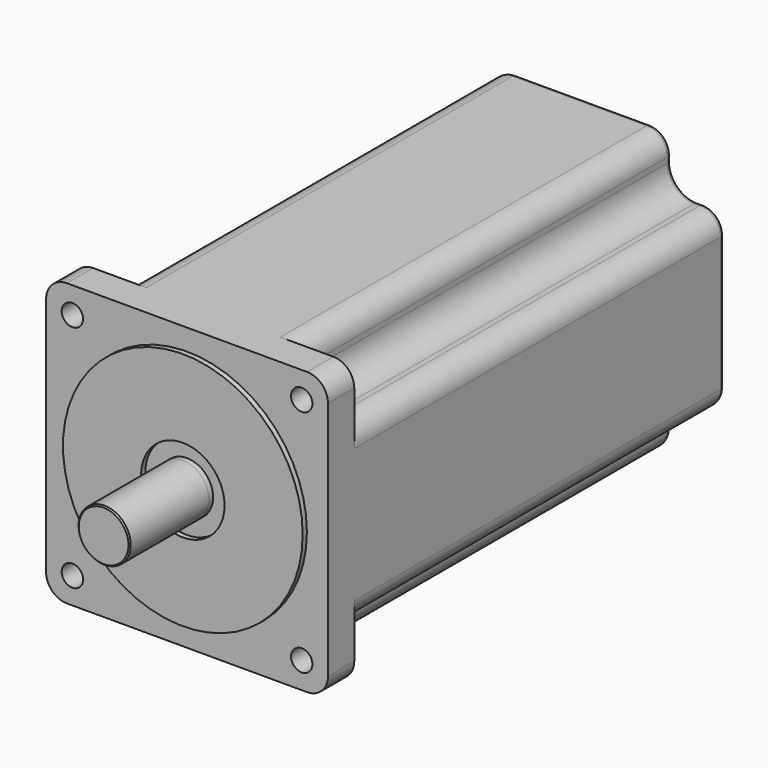
from build123d import *

# Parameters (mm, degrees)
F0_R         = 3.2512
F1_DEPTH     = 10.0076
F2_R         = 36.4998
F3_DEPTH     = 1.6002
F4_R         = 7.9375
F5_DEPTH     = 31.75
F6_SIZE      = 0.381
F7_R         = 12.7
F7_R_2       = 7.9375
F8_DEPTH     = 1.6002
F10_DEPTH    = 140.9954
F11_T1_DEPTH = 156.8704
F12_R        = 1.6002
F13_R        = 4.826
F14_DEPTH    = 12.7
F14_TAPER    = 1


# Not quite as in the source:
# - a fillet or chamfer that OpenCascade refuses, or shapes differently, is made with other operations: its cross-section is extruded or revolved along the edge and cut away or added


with BuildPart() as f1:
    # F0 (on Front) → F1 (new body)
    with BuildSketch(Plane.XZ):
        with BuildLine():
            ThreePointArc((42.926, 36.576), (41.0661280605, 41.0661280605), (36.576, 42.926))
            Line((36.576, 42.926), (-36.576, 42.926))
            ThreePointArc((-36.576, 42.926), (-41.0661280605, 41.0661280605), (-42.926, 36.576))
            Line((-42.926, 36.576), (-42.926, -36.576))
            ThreePointArc((-42.926, -36.576), (-41.0661280605, -41.0661280605), (-36.576, -42.926))
            Line((-36.576, -42.926), (36.576, -42.926))
            ThreePointArc((36.576, -42.926), (41.0661280605, -41.0661280605), (42.926, -36.576))
            Line((42.926, -36.576), (42.926, 36.576))
        make_face()
        with Locations((-34.925, -34.925)):
            Circle(F0_R, mode=Mode.SUBTRACT)
        with Locations((34.925, -34.925)):
            Circle(F0_R, mode=Mode.SUBTRACT)
        with Locations((-34.925, 34.925)):
            Circle(F0_R, mode=Mode.SUBTRACT)
        with Locations((34.925, 34.925)):
            Circle(F0_R, mode=Mode.SUBTRACT)
    extrude(amount=-F1_DEPTH)

    # F2 (on Front) → F3 (join)
    with BuildSketch(Plane.XZ):
        Circle(F2_R)
    extrude(amount=F3_DEPTH)

    # F4 (on Front) → F5 (join)
    with BuildSketch(Plane.XZ):
        Circle(F4_R)
    extrude(amount=F5_DEPTH)

    # F6
    f6_edges = [f1.edges().sort_by_distance(p)[0] for p in [
        (-7.9375, -31.75, 0),
    ]]
    chamfer(f6_edges, length=F6_SIZE)

    # F7 (on face) → F8 (cut)
    with BuildSketch(Plane.XZ.offset(1.6002)):
        Circle(F7_R)
        Circle(F7_R_2, mode=Mode.SUBTRACT)
    extrude(amount=-F8_DEPTH, mode=Mode.SUBTRACT)

    # F9 (on face) → F10 (join)
    with BuildSketch(Plane(origin=(0, 10.0076, 0), x_dir=(-1, 0, 0), z_dir=(0, 1, 0))):
        with BuildLine():
            ThreePointArc((-26.7554344057, 34.925), (-29.1482447689, 29.1482447689), (-34.925, 26.7554344057))
            Line((-34.925, 26.7554344057), (-42.926, 26.7554344057))
            Line((-42.926, 26.7554344057), (-42.926, -26.7554344057))
            Line((-42.926, -26.7554344057), (-34.925, -26.7554344057))
            ThreePointArc((-34.925, -26.7554344057), (-29.1482447689, -29.1482447689), (-26.7554344057, -34.925))
            Line((-26.7554344057, -34.925), (-26.7554344057, -42.926))
            Line((-26.7554344057, -42.926), (26.7554344057, -42.926))
            Line((26.7554344057, -42.926), (26.7554344057, -34.925))
            ThreePointArc((26.7554344057, -34.925), (29.1482447689, -29.1482447689), (34.925, -26.7554344057))
            Line((34.925, -26.7554344057), (42.926, -26.7554344057))
            Line((42.926, -26.7554344057), (42.926, 26.7554344057))
            Line((42.926, 26.7554344057), (34.925, 26.7554344057))
            ThreePointArc((34.925, 26.7554344057), (29.1482447689, 29.1482447689), (26.7554344057, 34.925))
            Line((26.7554344057, 34.925), (26.7554344057, 42.926))
            Line((26.7554344057, 42.926), (-26.7554344057, 42.926))
            Line((-26.7554344057, 42.926), (-26.7554344057, 34.925))
        make_face()
    extrude(amount=F10_DEPTH)

    # F11: fillet of radius 6.35 on 8 edges, made by hand

    # F11_s2 → F11_t1 (cut)
    with BuildSketch(Plane.XZ.offset(-166.878)):
        with BuildLine():
            ThreePointArc((20.4054344057, 42.926), (24.8955624662, 41.0661280605), (26.7554344057, 36.576))
            Line((26.7554344057, 36.576), (26.7554344057, 42.926))
            Line((26.7554344057, 42.926), (20.4054344057, 42.926))
        make_face()
        with BuildLine():
            ThreePointArc((42.926, 20.4054344057), (41.0661280605, 24.8955624662), (36.576, 26.7554344057))
            Line((36.576, 26.7554344057), (42.926, 26.7554344057))
            Line((42.926, 26.7554344057), (42.926, 20.4054344057))
        make_face()
        with BuildLine():
            ThreePointArc((42.926, -20.4054344057), (41.0661280605, -24.8955624662), (36.576, -26.7554344057))
            Line((36.576, -26.7554344057), (42.926, -26.7554344057))
            Line((42.926, -26.7554344057), (42.926, -20.4054344057))
        make_face()
        with BuildLine():
            ThreePointArc((20.4054344057, -42.926), (24.8955624662, -41.0661280605), (26.7554344057, -36.576))
            Line((26.7554344057, -36.576), (26.7554344057, -42.926))
            Line((26.7554344057, -42.926), (20.4054344057, -42.926))
        make_face()
        with BuildLine():
            ThreePointArc((-20.4054344057, 42.926), (-24.8955624662, 41.0661280605), (-26.7554344057, 36.576))
            Line((-26.7554344057, 36.576), (-26.7554344057, 42.926))
            Line((-26.7554344057, 42.926), (-20.4054344057, 42.926))
        make_face()
        with BuildLine():
            ThreePointArc((-42.926, 20.4054344057), (-41.0661280605, 24.8955624662), (-36.576, 26.7554344057))
            Line((-36.576, 26.7554344057), (-42.926, 26.7554344057))
            Line((-42.926, 26.7554344057), (-42.926, 20.4054344057))
        make_face()
        with BuildLine():
            ThreePointArc((-42.926, -20.4054344057), (-41.0661280605, -24.8955624662), (-36.576, -26.7554344057))
            Line((-36.576, -26.7554344057), (-42.926, -26.7554344057))
            Line((-42.926, -26.7554344057), (-42.926, -20.4054344057))
        make_face()
        with BuildLine():
            ThreePointArc((-20.4054344057, -42.926), (-24.8955624662, -41.0661280605), (-26.7554344057, -36.576))
            Line((-26.7554344057, -36.576), (-26.7554344057, -42.926))
            Line((-26.7554344057, -42.926), (-20.4054344057, -42.926))
        make_face()
    extrude(amount=F11_T1_DEPTH, mode=Mode.SUBTRACT)

    # F12
    f12_edges = [f1.edges().sort_by_distance(p)[0] for p in [
        (24.895562, 151.003, 41.066128),
    ]]
    fillet(f12_edges, radius=F12_R)

    # F13 (on face) → F14 (join)
    with BuildSketch(Plane(origin=(0, 0, -42.926), x_dir=(1, 0, 0), z_dir=(0, 0, -1))):
        with Locations((0, -136.7028)):
            Circle(F13_R)
    extrude(amount=F14_DEPTH, taper=F14_TAPER)


solid = f1.part
